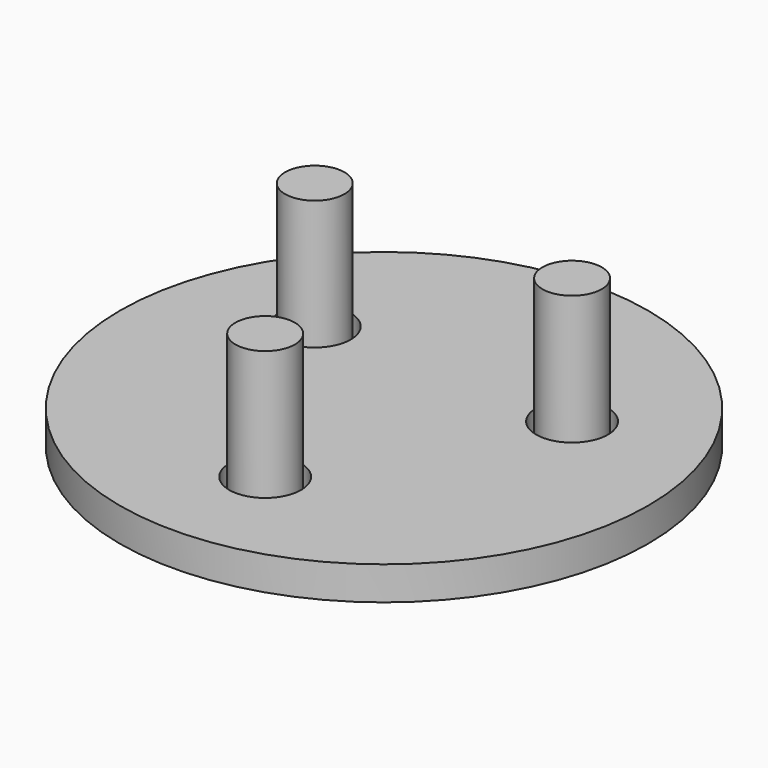
from build123d import *

# Parameters (mm, degrees)
F0_R     = 42.0452361361
F1_DEPTH = 5.334
F3_D     = 11.43
F2_R     = 4.7243980019
F4_DEPTH = 25.4


with BuildPart() as f1:
    # F0 (on Top) → F1 (new body)
    with BuildSketch(Plane.XY):
        Circle(F0_R)
    extrude(amount=F1_DEPTH)

    # F3 (through all)
    with Locations(Plane(origin=(0, 0, 0), x_dir=(1, 0, 0), z_dir=(0, 0, -1))):
        with Locations((-20.4800069598, -11.8241375312), (20.4800069598, -11.8241375312), (0, 23.6482750624)):
            Hole(F3_D / 2)


with BuildPart() as f4:
    # F2 (on Top) → F4 (new body)
    with BuildSketch(Plane.XY):
        with Locations((-20.4800069598, 11.8241375312)):
            Circle(F2_R)
    extrude(amount=F4_DEPTH)


with BuildPart() as f4b:
    # F2 (on Top) → F4, piece 2 (new body)
    with BuildSketch(Plane.XY):
        with Locations((20.4800069598, 11.8241375312)):
            Circle(F2_R)
    extrude(amount=F4_DEPTH)


with BuildPart() as f4c:
    # F2 (on Top) → F4, piece 3 (new body)
    with BuildSketch(Plane.XY):
        with Locations((0, -23.6482750624)):
            Circle(F2_R)
    extrude(amount=F4_DEPTH)


solid = Compound([f1.part, f4.part, f4b.part, f4c.part])
